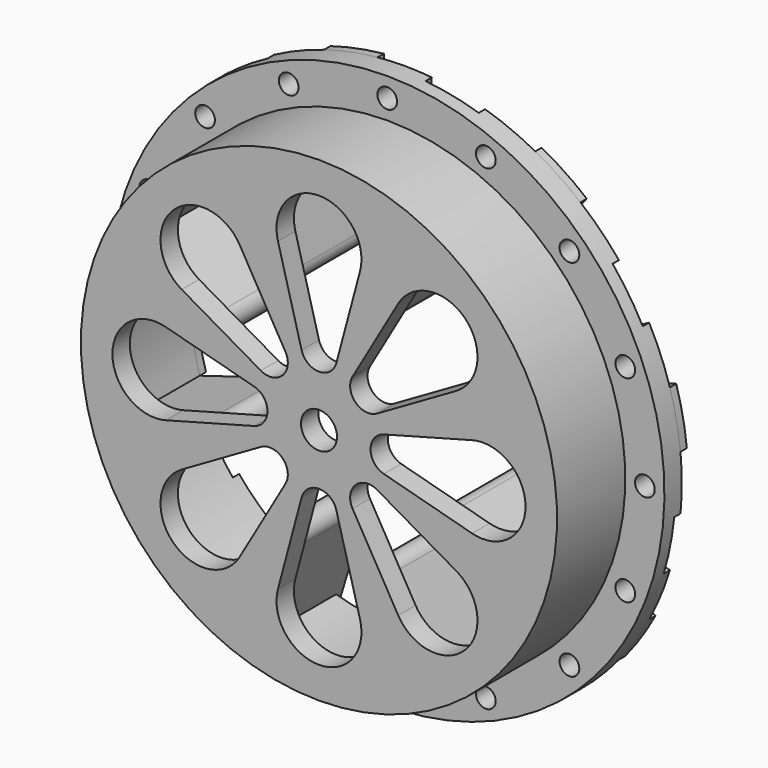
from build123d import *

# Parameters (mm, degrees)
F2_R          = 4.5662834284
F3_DEPTH      = 25
F3_DEPTH_BACK = 27.1704362164
F4_D          = 5
F9_DEPTH      = 21.652802825
F10_DEPTH     = 2
F11_DEPTH     = 2


with BuildPart() as f1:
    # F0 (on Right) → F1 (revolve)
    with BuildSketch(Plane.YZ):
        Polygon((-27.1694362164, 60.4071840644), (-27.1694362164, 0), (-21.652802825, 0), (-21.652802825, 54.3388873339), (0, 54.3388873339), (0, 70.3371316195), (-5.5166333914, 70.3371316195), (-5.5166333914, 60.4071840644), align=None)
    revolve(axis=Axis((0, -24.4111195207, 0), (0, -1, 0)))

    # F2 (on Front) → F3 (cut, two sides)
    with BuildSketch(Plane.XZ) as f3_sk:
        with BuildLine():
            ThreePointArc((-4.4106910937, 16.460923258), (0, 13.0764809462), (4.4106910937, 16.460923258))
            Line((4.4106910937, 16.460923258), (10.408250615, 38.8441201131))
            ThreePointArc((10.408250615, 38.8441201131), (0, 52.4084164015), (-10.408250615, 38.8441201131))
            Line((-10.408250615, 38.8441201131), (-4.4106910937, 16.460923258))
        make_face()
        with BuildLine():
            Line((-8.5208008783, 14.7584600424), (-20.107196151, 34.8266853313))
            ThreePointArc((-20.107196151, 34.8266853313), (-37.0583466287, 37.0583466287), (-34.8266853313, 20.107196151))
            Line((-34.8266853313, 20.107196151), (-14.7584600424, 8.5208008783))
            ThreePointArc((-14.7584600424, 8.5208008783), (-9.2464683511, 9.2464683511), (-8.5208008783, 14.7584600424))
        make_face()
        with BuildLine():
            Line((-16.460923258, 4.4106910937), (-38.8441201131, 10.408250615))
            ThreePointArc((-38.8441201131, 10.408250615), (-52.4084164015, 0), (-38.8441201131, -10.408250615))
            Line((-38.8441201131, -10.408250615), (-16.460923258, -4.4106910937))
            ThreePointArc((-16.460923258, -4.4106910937), (-13.0764809462, 0), (-16.460923258, 4.4106910937))
        make_face()
        with BuildLine():
            Line((-14.7584600424, -8.5208008783), (-34.8266853313, -20.107196151))
            ThreePointArc((-34.8266853313, -20.107196151), (-37.0583466287, -37.0583466287), (-20.107196151, -34.8266853313))
            Line((-20.107196151, -34.8266853313), (-8.5208008783, -14.7584600424))
            ThreePointArc((-8.5208008783, -14.7584600424), (-9.2464683511, -9.2464683511), (-14.7584600424, -8.5208008783))
        make_face()
        with BuildLine():
            Line((-4.4106910937, -16.460923258), (-10.408250615, -38.8441201131))
            ThreePointArc((-10.408250615, -38.8441201131), (0, -52.4084164015), (10.408250615, -38.8441201131))
            Line((10.408250615, -38.8441201131), (4.4106910937, -16.460923258))
            ThreePointArc((4.4106910937, -16.460923258), (0, -13.0764809462), (-4.4106910937, -16.460923258))
        make_face()
        with BuildLine():
            Line((8.5208008783, -14.7584600424), (20.107196151, -34.8266853313))
            ThreePointArc((20.107196151, -34.8266853313), (37.0583466287, -37.0583466287), (34.8266853313, -20.107196151))
            Line((34.8266853313, -20.107196151), (14.7584600424, -8.5208008783))
            ThreePointArc((14.7584600424, -8.5208008783), (9.2464683511, -9.2464683511), (8.5208008783, -14.7584600424))
        make_face()
        Circle(F2_R)
        with BuildLine():
            Line((16.460923258, -4.4106910937), (38.8441201131, -10.408250615))
            ThreePointArc((38.8441201131, -10.408250615), (52.4084164015, 0), (38.8441201131, 10.408250615))
            Line((38.8441201131, 10.408250615), (16.460923258, 4.4106910937))
            ThreePointArc((16.460923258, 4.4106910937), (13.0764809462, 0), (16.460923258, -4.4106910937))
        make_face()
        with BuildLine():
            Line((14.7584600424, 8.5208008783), (34.8266853313, 20.107196151))
            ThreePointArc((34.8266853313, 20.107196151), (37.0583466287, 37.0583466287), (20.107196151, 34.8266853313))
            Line((20.107196151, 34.8266853313), (8.5208008783, 14.7584600424))
            ThreePointArc((8.5208008783, 14.7584600424), (9.2464683511, 9.2464683511), (14.7584600424, 8.5208008783))
        make_face()
    extrude(amount=-F3_DEPTH, mode=Mode.SUBTRACT)
    extrude(f3_sk.sketch, amount=F3_DEPTH_BACK, mode=Mode.SUBTRACT)

    # F4 (through all)
    with Locations(Plane(origin=(0, 0, 0), x_dir=(1, 0, 0), z_dir=(0, 1, 0))):
        with Locations((0, -65.3721578419), (-25.0168417441, -60.3959986262), (-46.2250961108, -46.2250961108), (-60.3959986262, -25.0168417441), (-65.3721578419, 0), (-60.3959986262, 25.0168417441), (-46.2250961108, 46.2250961108), (-25.0168417441, 60.3959986262), (0, 65.3721578419), (25.0168417441, 60.3959986262), (46.2250961108, 46.2250961108), (60.3959986262, 25.0168417441), (65.3721578419, 0), (60.3959986262, -25.0168417441), (46.2250961108, -46.2250961108), (25.0168417441, -60.3959986262)):
            Hole(F4_D / 2)

    # F6 (on face) → F9 (join, through all)
    with BuildSketch(Plane.XZ):
        with BuildLine():
            ThreePointArc((9.4425792671, 31.1280121965), (11.2823812281, 27.2380777768), (15.3339166773, 28.6877403406))
            Line((15.3339166773, 28.6877403406), (25.6151741719, 47.9226202208))
            ThreePointArc((25.6151741719, 47.9226202208), (20.7945919158, 50.2025858272), (15.7737463721, 51.9990730886))
            Line((15.7737463721, 51.9990730886), (9.4425792671, 31.1280121965))
        make_face()
        with BuildLine():
            Line((-9.4425792671, 31.1280121965), (-15.7737463721, 51.9990730886))
            ThreePointArc((-15.7737463721, 51.9990730886), (-20.7945919158, 50.2025858272), (-25.6151741719, 47.9226202208))
            Line((-25.6151741719, 47.9226202208), (-15.3339166773, 28.6877403406))
            ThreePointArc((-15.3339166773, 28.6877403406), (-11.2823812281, 27.2380777768), (-9.4425792671, 31.1280121965))
        make_face()
        with BuildLine():
            Line((-28.6877403406, 15.3339166773), (-47.9226202208, 25.6151741719))
            ThreePointArc((-47.9226202208, 25.6151741719), (-50.2025858272, 20.7945919158), (-51.9990730886, 15.7737463721))
            Line((-51.9990730886, 15.7737463721), (-31.1280121965, 9.4425792671))
            ThreePointArc((-31.1280121965, 9.4425792671), (-27.2380777768, 11.2823812281), (-28.6877403406, 15.3339166773))
        make_face()
        with BuildLine():
            Line((-31.1280121965, -9.4425792671), (-51.9990730886, -15.7737463721))
            ThreePointArc((-51.9990730886, -15.7737463721), (-50.2025858272, -20.7945919158), (-47.9226202208, -25.6151741719))
            Line((-47.9226202208, -25.6151741719), (-28.6877403406, -15.3339166773))
            ThreePointArc((-28.6877403406, -15.3339166773), (-27.2380777768, -11.2823812281), (-31.1280121965, -9.4425792671))
        make_face()
        with BuildLine():
            Line((-15.3339166773, -28.6877403406), (-25.6151741719, -47.9226202208))
            ThreePointArc((-25.6151741719, -47.9226202208), (-20.7945919158, -50.2025858272), (-15.7737463721, -51.9990730886))
            Line((-15.7737463721, -51.9990730886), (-9.4425792671, -31.1280121965))
            ThreePointArc((-9.4425792671, -31.1280121965), (-11.2823812281, -27.2380777768), (-15.3339166773, -28.6877403406))
        make_face()
        with BuildLine():
            Line((9.4425792671, -31.1280121965), (15.7737463721, -51.9990730886))
            ThreePointArc((15.7737463721, -51.9990730886), (20.7945919158, -50.2025858272), (25.6151741719, -47.9226202208))
            Line((25.6151741719, -47.9226202208), (15.3339166773, -28.6877403406))
            ThreePointArc((15.3339166773, -28.6877403406), (11.2823812281, -27.2380777768), (9.4425792671, -31.1280121965))
        make_face()
        with BuildLine():
            Line((28.6877403406, -15.3339166773), (47.9226202208, -25.6151741719))
            ThreePointArc((47.9226202208, -25.6151741719), (50.2025858272, -20.7945919158), (51.9990730886, -15.7737463721))
            Line((51.9990730886, -15.7737463721), (31.1280121965, -9.4425792671))
            ThreePointArc((31.1280121965, -9.4425792671), (27.2380777768, -11.2823812281), (28.6877403406, -15.3339166773))
        make_face()
        with BuildLine():
            Line((31.1280121965, 9.4425792671), (51.9990730886, 15.7737463721))
            ThreePointArc((51.9990730886, 15.7737463721), (50.2025858272, 20.7945919158), (47.9226202208, 25.6151741719))
            Line((47.9226202208, 25.6151741719), (28.6877403406, 15.3339166773))
            ThreePointArc((28.6877403406, 15.3339166773), (27.2380777768, 11.2823812281), (31.1280121965, 9.4425792671))
        make_face()
    extrude(amount=F9_DEPTH)

    # F7 (on face) → F10 (cut)
    with BuildSketch(Plane.XZ):
        with BuildLine():
            ThreePointArc((5.3261423452, 54.077230739), (10.600991028, 53.2947808505), (15.7737463721, 51.9990730886))
            Line((15.7737463721, 51.9990730886), (20.4177915512, 67.3084383464))
            ThreePointArc((20.4177915512, 67.3084383464), (13.7220936573, 68.9856233581), (6.8942445003, 69.9984391056))
            Line((6.8942445003, 69.9984391056), (5.3261423452, 54.077230739))
        make_face()
        with BuildLine():
            ThreePointArc((-33.1566943231, 62.0318120485), (-39.0772166038, 58.4831875581), (-44.6214039267, 54.3713380014))
            Line((-44.6214039267, 54.3713380014), (-34.4722251935, 42.0045279332))
            ThreePointArc((-34.4722251935, 42.0045279332), (-30.1890682981, 45.1811335844), (-25.6151741719, 47.9226202208))
            Line((-25.6151741719, 47.9226202208), (-33.1566943231, 62.0318120485))
        make_face()
        with BuildLine():
            ThreePointArc((-67.3084383464, 20.4177915512), (-68.9856233581, 13.7220936573), (-69.9984391056, 6.8942445003))
            Line((-69.9984391056, 6.8942445003), (-54.077230739, 5.3261423452))
            ThreePointArc((-54.077230739, 5.3261423452), (-53.2947808505, 10.600991028), (-51.9990730886, 15.7737463721))
            Line((-51.9990730886, 15.7737463721), (-67.3084383464, 20.4177915512))
        make_face()
        with BuildLine():
            ThreePointArc((-62.0318120485, -33.1566943231), (-58.4831875581, -39.0772166038), (-54.3713380014, -44.6214039267))
            Line((-54.3713380014, -44.6214039267), (-42.0045279332, -34.4722251935))
            ThreePointArc((-42.0045279332, -34.4722251935), (-45.1811335844, -30.1890682981), (-47.9226202208, -25.6151741719))
            Line((-47.9226202208, -25.6151741719), (-62.0318120485, -33.1566943231))
        make_face()
        with BuildLine():
            ThreePointArc((-20.4177915512, -67.3084383464), (-13.7220936573, -68.9856233581), (-6.8942445003, -69.9984391056))
            Line((-6.8942445003, -69.9984391056), (-5.3261423452, -54.077230739))
            ThreePointArc((-5.3261423452, -54.077230739), (-10.600991028, -53.2947808505), (-15.7737463721, -51.9990730886))
            Line((-15.7737463721, -51.9990730886), (-20.4177915512, -67.3084383464))
        make_face()
        with BuildLine():
            ThreePointArc((33.1566943231, -62.0318120485), (39.0772166038, -58.4831875581), (44.6214039267, -54.3713380014))
            Line((44.6214039267, -54.3713380014), (34.4722251935, -42.0045279332))
            ThreePointArc((34.4722251935, -42.0045279332), (30.1890682981, -45.1811335844), (25.6151741719, -47.9226202208))
            Line((25.6151741719, -47.9226202208), (33.1566943231, -62.0318120485))
        make_face()
        with BuildLine():
            ThreePointArc((67.3084383464, -20.4177915512), (68.9856233581, -13.7220936573), (69.9984391056, -6.8942445003))
            Line((69.9984391056, -6.8942445003), (54.077230739, -5.3261423452))
            ThreePointArc((54.077230739, -5.3261423452), (53.2947808505, -10.600991028), (51.9990730886, -15.7737463721))
            Line((51.9990730886, -15.7737463721), (67.3084383464, -20.4177915512))
        make_face()
        with BuildLine():
            ThreePointArc((62.0318120485, 33.1566943231), (58.4831875581, 39.0772166038), (54.3713380014, 44.6214039267))
            Line((54.3713380014, 44.6214039267), (42.0045279332, 34.4722251935))
            ThreePointArc((42.0045279332, 34.4722251935), (45.1811335844, 30.1890682981), (47.9226202208, 25.6151741719))
            Line((47.9226202208, 25.6151741719), (62.0318120485, 33.1566943231))
        make_face()
    extrude(amount=F10_DEPTH, mode=Mode.SUBTRACT)

    # F8 (on face) → F11 (join)
    with BuildSketch(Plane.XZ):
        with BuildLine():
            ThreePointArc((44.6214039267, 54.3713380014), (39.0772166038, 58.4831875581), (33.1566943231, 62.0318120485))
            Line((33.1566943231, 62.0318120485), (25.6151741719, 47.9226202208))
            ThreePointArc((25.6151741719, 47.9226202208), (30.1890682981, 45.1811335844), (34.4722251935, 42.0045279332))
            Line((34.4722251935, 42.0045279332), (44.6214039267, 54.3713380014))
        make_face()
        with BuildLine():
            ThreePointArc((-6.8942445003, 69.9984391056), (-13.7220936573, 68.9856233581), (-20.4177915512, 67.3084383464))
            Line((-20.4177915512, 67.3084383464), (-15.7737463721, 51.9990730886))
            ThreePointArc((-15.7737463721, 51.9990730886), (-10.600991028, 53.2947808505), (-5.3261423452, 54.077230739))
            Line((-5.3261423452, 54.077230739), (-6.8942445003, 69.9984391056))
        make_face()
        with BuildLine():
            ThreePointArc((-54.3713380014, 44.6214039267), (-58.4831875581, 39.0772166038), (-62.0318120485, 33.1566943231))
            Line((-62.0318120485, 33.1566943231), (-47.9226202208, 25.6151741719))
            ThreePointArc((-47.9226202208, 25.6151741719), (-45.1811335844, 30.1890682981), (-42.0045279332, 34.4722251935))
            Line((-42.0045279332, 34.4722251935), (-54.3713380014, 44.6214039267))
        make_face()
        with BuildLine():
            ThreePointArc((-69.9984391056, -6.8942445003), (-68.9856233581, -13.7220936573), (-67.3084383464, -20.4177915512))
            Line((-67.3084383464, -20.4177915512), (-51.9990730886, -15.7737463721))
            ThreePointArc((-51.9990730886, -15.7737463721), (-53.2947808505, -10.600991028), (-54.077230739, -5.3261423452))
            Line((-54.077230739, -5.3261423452), (-69.9984391056, -6.8942445003))
        make_face()
        with BuildLine():
            ThreePointArc((-44.6214039267, -54.3713380014), (-39.0772166038, -58.4831875581), (-33.1566943231, -62.0318120485))
            Line((-33.1566943231, -62.0318120485), (-25.6151741719, -47.9226202208))
            ThreePointArc((-25.6151741719, -47.9226202208), (-30.1890682981, -45.1811335844), (-34.4722251935, -42.0045279332))
            Line((-34.4722251935, -42.0045279332), (-44.6214039267, -54.3713380014))
        make_face()
        with BuildLine():
            ThreePointArc((6.8942445003, -69.9984391056), (13.7220936573, -68.9856233581), (20.4177915512, -67.3084383464))
            Line((20.4177915512, -67.3084383464), (15.7737463721, -51.9990730886))
            ThreePointArc((15.7737463721, -51.9990730886), (10.600991028, -53.2947808505), (5.3261423452, -54.077230739))
            Line((5.3261423452, -54.077230739), (6.8942445003, -69.9984391056))
        make_face()
        with BuildLine():
            ThreePointArc((54.3713380014, -44.6214039267), (58.4831875581, -39.0772166038), (62.0318120485, -33.1566943231))
            Line((62.0318120485, -33.1566943231), (47.9226202208, -25.6151741719))
            ThreePointArc((47.9226202208, -25.6151741719), (45.1811335844, -30.1890682981), (42.0045279332, -34.4722251935))
            Line((42.0045279332, -34.4722251935), (54.3713380014, -44.6214039267))
        make_face()
        with BuildLine():
            ThreePointArc((69.9984391056, 6.8942445003), (68.9856233581, 13.7220936573), (67.3084383464, 20.4177915512))
            Line((67.3084383464, 20.4177915512), (51.9990730886, 15.7737463721))
            ThreePointArc((51.9990730886, 15.7737463721), (53.2947808505, 10.600991028), (54.077230739, 5.3261423452))
            Line((54.077230739, 5.3261423452), (69.9984391056, 6.8942445003))
        make_face()
    extrude(amount=-F11_DEPTH)


solid = f1.part
